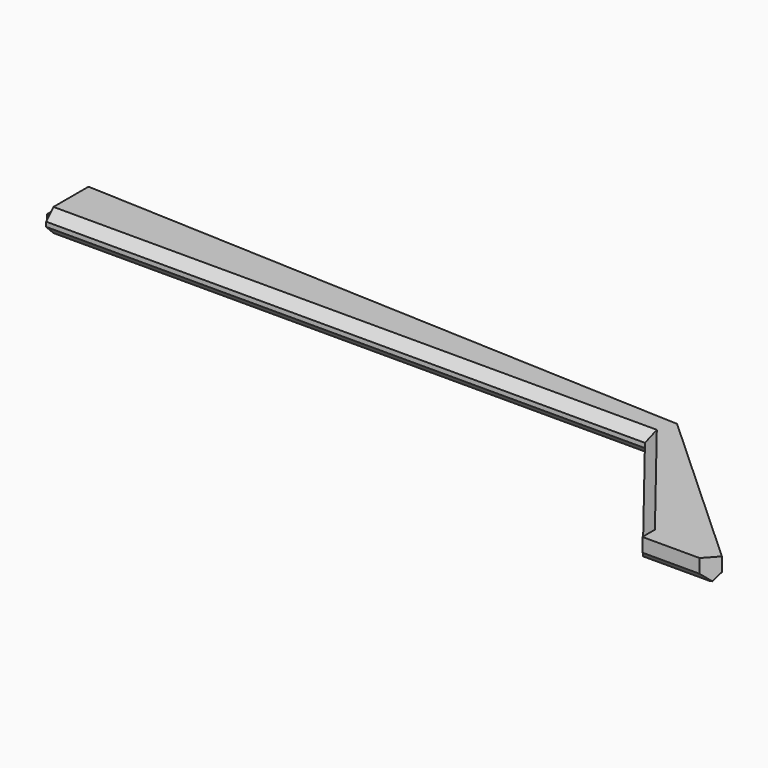
from build123d import *

# Parameters (mm, degrees)
F1_DEPTH = 5
F2_SIZE  = 2
F0_W     = 2.8
F0_H     = 9.8
F3_DEPTH = 2


# Not quite as in the source:
# - a feature of the source that left no trace in its solid (it failed there, or was rolled back) is left out


with BuildPart() as f1:
    # F0 (on Top) → F1 (new body)
    with BuildSketch(Plane.XY):
        Polygon((49.7136654785, 23.7398390386), (-80.2863345215, 29.3157004521), (-80.2863345215, 19.5157004521), (-80.2863345215, 15.7984595098), (49.7136654785, 15.7984595098), (73.3425258757, -14.2773987355), (73.3425258757, -14.4394316876), (85.7469019117, -14.4394316876), (88.3425258757, -11.6024324968), align=None)
    extrude(amount=F1_DEPTH)

    # F2 (call 1 of 5: OpenCascade refuses the feature's edges together)
    f2_edges = [f1.edges().sort_by_distance(p)[0] for p in [
        (-15.286335, 15.79846, 0),
    ]]
    chamfer(f2_edges, length=F2_SIZE)

    # F2#2 (call 2 of 5)
    f2_2_edges = [f1.edges().sort_by_distance(p)[0] for p in [
        (69.028096, 6.068703, 0),
    ]]
    chamfer(f2_2_edges, length=F2_SIZE)

    # F2#3 (call 3 of 5)
    f2_3_edges = [f1.edges().sort_by_distance(p)[0] for p in [
        (79.544714, -14.439432, 0),
    ]]
    chamfer(f2_3_edges, length=F2_SIZE)

    # F2#4 (call 4 of 5)
    f2_4_edges = [f1.edges().sort_by_distance(p)[0] for p in [
        (61.528096, 0.76053, 5),
        (-15.286335, 15.79846, 5),
    ]]
    chamfer(f2_4_edges, length=F2_SIZE)

    # F2#5 (call 5 of 5)
    f2_5_edges = [f1.edges().sort_by_distance(p)[0] for p in [
        (-15.286335, 26.52777, 5),
    ]]
    chamfer(f2_5_edges, length=F2_SIZE)

    # F0 (on Top) → F3 (join)
    with BuildSketch(Plane.XY):
        with Locations((-81.6863345215, 24.4157004521)):
            Rectangle(F0_W, F0_H)
    extrude(amount=F3_DEPTH)


solid = f1.part
